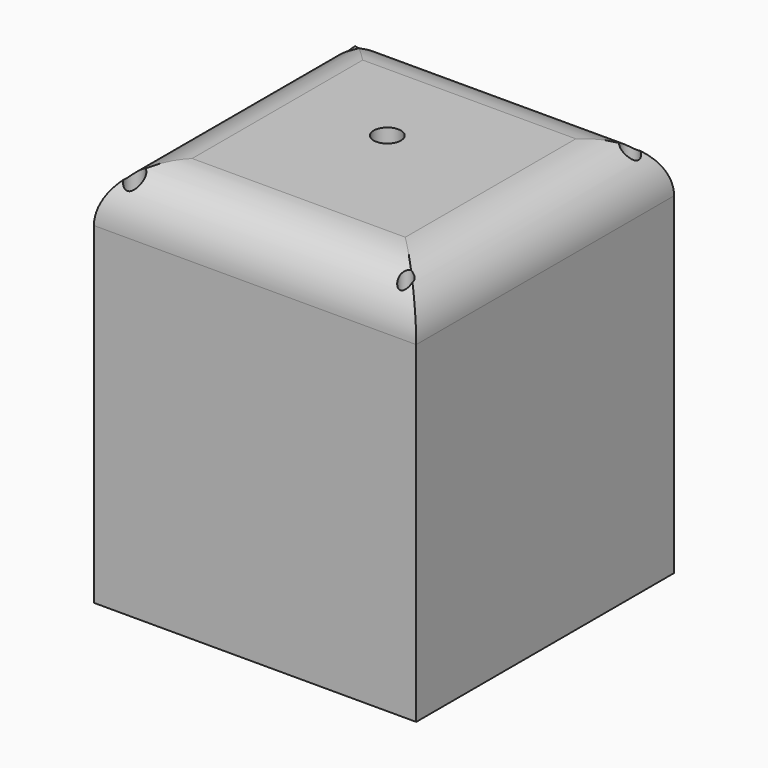
from build123d import *

# Parameters (mm, degrees)
F0_W         = 60
F0_H         = 60
F0_R         = 4
F0_R_2       = 2.5
F0_R_3       = 3.4946911037
F0_R_4       = 3.5
F1_DEPTH     = 50
F2_T1_DEPTH  = 75.4
F2_T3_DEPTH  = 25.2382554531
F2_T5_DEPTH  = 27.4689431906
F2_T7_DEPTH  = 23.1458252341
F2_T9_DEPTH  = 24.307484892
F3_W         = 60
F3_H         = 60
F3_W_2       = 50.3480000794
F3_H_2       = 50.3480000794
F4_DEPTH     = 20
F5_W         = 60
F5_H         = 60
F6_DEPTH     = 2
F7_R         = 5.1102202796
F8_DEPTH     = 70
F9_T1_DEPTH  = 50.3480000794
F9_T3_DEPTH  = 50.3480000794
F9_T7_DEPTH  = 110.8
F9_T9_DEPTH  = 110.8
F10_T1_DEPTH = 69.9999999998
F10_T4_ANGLE = 90
F11_T1_DEPTH = 69.9999999998
F11_T4_ANGLE = 90
F12_T1_DEPTH = 69.9999999998
F12_T4_ANGLE = 90
F13_T1_DEPTH = 24.2745776091
F13_T3_DEPTH = 45.7254223907
F13_T6_ANGLE = 90
F14_R        = 1.700912826
F14_R_2      = 1.2677188497
F14_R_3      = 1.5887309538
F14_R_4      = 2.5350136115
F15_DEPTH    = 72.001
F16_R        = 2.5348197432
F17_DEPTH    = 72.0010001


# Not quite as in the source:
# - a fillet or chamfer that OpenCascade refuses, or shapes differently, is made with other operations: its cross-section is extruded or revolved along the edge and cut away or added


with BuildPart() as f1:
    # F0 (on Top) → F1 (new body)
    with BuildSketch(Plane.XY):
        with Locations((-30, 30)):
            Rectangle(F0_W, F0_H)
        with Locations((-31.7886509001, 10.1095326245)):
            Circle(F0_R, mode=Mode.SUBTRACT)
        with Locations((-48.9362515509, 26.676196605)):
            Circle(F0_R_2, mode=Mode.SUBTRACT)
        Polygon((-4.8259999603, 24.6461443603), (-4.8259999603, 4.8259999603), (-22.2616568208, 4.8259999603), (-22.2616568208, 16.4334848523), (-39.9156734347, 16.4334848523), (-39.9156734347, 4.8259999603), (-55.1740000397, 4.8259999603), (-55.1740000397, 22.681651637), (-43.3133915067, 22.681651637), (-43.3133915067, 30), (-55.1740000397, 30), (-55.1740000397, 55.1740000397), (-42.5382554531, 55.1740000397), (-42.5382554531, 44.7281748056), (-30, 44.7281748056), (-30, 55.1740000397), (-4.8259999603, 55.1740000397), (-4.8259999603, 37.5920906663), (-19.5949431509, 37.5920906663), (-19.5949431509, 24.6461443603), align=None, mode=Mode.SUBTRACT)
        with Locations((-36.420982331, 50.7049895823)):
            Circle(F0_R_3, mode=Mode.SUBTRACT)
        with Locations((-12.2104715556, 31.8728536367)):
            Circle(F0_R_4, mode=Mode.SUBTRACT)
    extrude(amount=F1_DEPTH)

    # F2: fillet of radius 5.08 on 13 edges, made by hand

    # F2_s2 → F2_t1 (cut)
    with BuildSketch(Plane.XY.offset(-12.7)):
        with BuildLine():
            ThreePointArc((-43.3133915067, 24.92), (-44.8012890582, 28.5121024484), (-48.3933915067, 30))
            Line((-48.3933915067, 30), (-43.3133915067, 30))
            Line((-43.3133915067, 30), (-43.3133915067, 24.92))
        make_face()
        with BuildLine():
            ThreePointArc((-48.3933915067, 22.681651637), (-44.8012890582, 24.1695491885), (-43.3133915067, 27.761651637))
            Line((-43.3133915067, 27.761651637), (-43.3133915067, 22.681651637))
            Line((-43.3133915067, 22.681651637), (-48.3933915067, 22.681651637))
        make_face()
        with BuildLine():
            ThreePointArc((-19.5949431509, 29.7261443603), (-18.1070455993, 26.1340419119), (-14.5149431509, 24.6461443603))
            Line((-14.5149431509, 24.6461443603), (-19.5949431509, 24.6461443603))
            Line((-19.5949431509, 24.6461443603), (-19.5949431509, 29.7261443603))
        make_face()
        with BuildLine():
            ThreePointArc((-14.5149431509, 37.5920906663), (-18.1070455993, 36.1041931147), (-19.5949431509, 32.5120906663))
            Line((-19.5949431509, 32.5120906663), (-19.5949431509, 37.5920906663))
            Line((-19.5949431509, 37.5920906663), (-14.5149431509, 37.5920906663))
        make_face()
        with BuildLine():
            ThreePointArc((-34.8356734347, 16.4334848523), (-38.4277758832, 14.9455873007), (-39.9156734347, 11.3534848523))
            Line((-39.9156734347, 11.3534848523), (-39.9156734347, 16.4334848523))
            Line((-39.9156734347, 16.4334848523), (-34.8356734347, 16.4334848523))
        make_face()
        with BuildLine():
            ThreePointArc((-22.2616568208, 11.3534848523), (-23.7495543723, 14.9455873007), (-27.3416568208, 16.4334848523))
            Line((-27.3416568208, 16.4334848523), (-22.2616568208, 16.4334848523))
            Line((-22.2616568208, 16.4334848523), (-22.2616568208, 11.3534848523))
        make_face()
    extrude(amount=F2_T1_DEPTH, mode=Mode.SUBTRACT)

    # F2_s4 → F2_t3 (cut)
    with BuildSketch(Plane.YZ.offset(-42.5382554531)):
        with BuildLine():
            ThreePointArc((44.7281748056, 44.92), (46.2160723572, 48.5121024484), (49.8081748056, 50))
            Line((49.8081748056, 50), (44.7281748056, 50))
            Line((44.7281748056, 50), (44.7281748056, 44.92))
        make_face()
    extrude(amount=F2_T3_DEPTH, mode=Mode.SUBTRACT)

    # F2_s6 → F2_t5 (cut)
    with BuildSketch(Plane.YZ.offset(-32.2949431509)):
        with BuildLine():
            ThreePointArc((37.5920906663, 44.92), (36.1041931147, 48.5121024484), (32.5120906663, 50))
            Line((32.5120906663, 50), (37.5920906663, 50))
            Line((37.5920906663, 50), (37.5920906663, 44.92))
        make_face()
        with BuildLine():
            ThreePointArc((24.6461443603, 44.92), (26.1340419119, 48.5121024484), (29.7261443603, 50))
            Line((29.7261443603, 50), (24.6461443603, 50))
            Line((24.6461443603, 50), (24.6461443603, 44.92))
        make_face()
    extrude(amount=F2_T5_DEPTH, mode=Mode.SUBTRACT)

    # F2_s8 → F2_t7 (cut)
    with BuildSketch(Plane.XZ.offset(-55.1740000397)):
        with BuildLine():
            ThreePointArc((-42.5382554531, 44.92), (-41.0503579015, 48.5121024484), (-37.4582554531, 50))
            Line((-37.4582554531, 50), (-42.5382554531, 50))
            Line((-42.5382554531, 50), (-42.5382554531, 44.92))
        make_face()
        with BuildLine():
            ThreePointArc((-30, 44.92), (-31.4878975516, 48.5121024484), (-35.08, 50))
            Line((-35.08, 50), (-30, 50))
            Line((-30, 50), (-30, 44.92))
        make_face()
    extrude(amount=F2_T7_DEPTH, mode=Mode.SUBTRACT)

    # F2_s10 → F2_t9 (cut)
    with BuildSketch(Plane.XZ.offset(-29.1334848523)):
        with BuildLine():
            ThreePointArc((-22.2616568208, 44.92), (-23.7495543723, 48.5121024484), (-27.3416568208, 50))
            Line((-27.3416568208, 50), (-22.2616568208, 50))
            Line((-22.2616568208, 50), (-22.2616568208, 44.92))
        make_face()
        with BuildLine():
            ThreePointArc((-39.9156734347, 44.92), (-38.4277758832, 48.5121024484), (-34.8356734347, 50))
            Line((-34.8356734347, 50), (-39.9156734347, 50))
            Line((-39.9156734347, 50), (-39.9156734347, 44.92))
        make_face()
    extrude(amount=F2_T9_DEPTH, mode=Mode.SUBTRACT)

    # F3 (on face) → F4 (join)
    with BuildSketch(Plane.XY.offset(50)):
        with Locations((-30, 30)):
            Rectangle(F3_W, F3_H)
        with Locations((-30, 30)):
            Rectangle(F3_W_2, F3_H_2, mode=Mode.SUBTRACT)
    extrude(amount=F4_DEPTH)

    # F5 (on face) → F6 (join)
    with BuildSketch(Plane.XY.offset(70)):
        with Locations((-30, 30)):
            Rectangle(F5_W, F5_H)
    extrude(amount=F6_DEPTH)

    # F7 (on Top) → F8 (join)
    with BuildSketch(Plane.XY):
        with Locations((-32.2121977806, 33.5347950459)):
            Circle(F7_R)
    extrude(amount=F8_DEPTH)

    # F9: fillet of radius 10.16 on 9 edges, made by hand

    # F9_s2 → F9_t1 (join)
    with BuildSketch(Plane.XZ.offset(-55.1740000397)):
        with BuildLine():
            ThreePointArc((-4.8259999603, 59.84), (-7.8017950634, 67.0242048969), (-14.9859999603, 70))
            Line((-14.9859999603, 70), (-4.8259999603, 70))
            Line((-4.8259999603, 70), (-4.8259999603, 59.84))
        make_face()
        with BuildLine():
            ThreePointArc((-55.1740000397, 59.84), (-52.1982049366, 67.0242048969), (-45.0140000397, 70))
            Line((-45.0140000397, 70), (-55.1740000397, 70))
            Line((-55.1740000397, 70), (-55.1740000397, 59.84))
        make_face()
    extrude(amount=F9_T1_DEPTH)

    # F9_s4 → F9_t3 (join)
    with BuildSketch(Plane.YZ.offset(-55.1740000397)):
        with BuildLine():
            ThreePointArc((4.8259999603, 59.84), (7.8017950634, 67.0242048969), (14.9859999603, 70))
            Line((14.9859999603, 70), (4.8259999603, 70))
            Line((4.8259999603, 70), (4.8259999603, 59.84))
        make_face()
        with BuildLine():
            ThreePointArc((55.1740000397, 59.84), (52.1982049366, 67.0242048969), (45.0140000397, 70))
            Line((45.0140000397, 70), (55.1740000397, 70))
            Line((55.1740000397, 70), (55.1740000397, 59.84))
        make_face()
    extrude(amount=F9_T3_DEPTH)

    # F9_s5 → F9_t6 (revolve)
    with BuildSketch(Plane.XZ.offset(-33.5347950459)):
        with BuildLine():
            ThreePointArc((-16.941977501, 70), (-24.1261823978, 67.0242048969), (-27.101977501, 59.84))
            Line((-27.101977501, 59.84), (-27.101977501, 70))
            Line((-27.101977501, 70), (-16.941977501, 70))
        make_face()
    revolve(axis=Axis((-32.2121977806, 33.5347950459, 70), (0, 0, 1)))

    # F9_s8 → F9_t7 (cut)
    with BuildSketch(Plane.XZ.offset(-85.4)):
        with BuildLine():
            ThreePointArc((-10.16, 72), (-2.9757951031, 69.0242048969), (0, 61.84))
            Line((0, 61.84), (0, 72))
            Line((0, 72), (-10.16, 72))
        make_face()
        with BuildLine():
            ThreePointArc((-60, 61.84), (-57.0242048969, 69.0242048969), (-49.84, 72))
            Line((-49.84, 72), (-60, 72))
            Line((-60, 72), (-60, 61.84))
        make_face()
    extrude(amount=F9_T7_DEPTH, mode=Mode.SUBTRACT)

    # F9_s10 → F9_t9 (cut)
    with BuildSketch(Plane.YZ.offset(-85.4)):
        with BuildLine():
            ThreePointArc((49.84, 72), (57.0242048969, 69.0242048969), (60, 61.84))
            Line((60, 61.84), (60, 72))
            Line((60, 72), (49.84, 72))
        make_face()
        with BuildLine():
            ThreePointArc((0, 61.84), (2.9757951031, 69.0242048969), (10.16, 72))
            Line((10.16, 72), (0, 72))
            Line((0, 72), (0, 61.84))
        make_face()
    extrude(amount=F9_T9_DEPTH, mode=Mode.SUBTRACT)

    # F10: fillet of radius 12.7 on 1 edges, made by hand

    # F10_s2 → F10_t1 (join)
    with BuildSketch(Plane.XY):
        with BuildLine():
            ThreePointArc((-55.1740000397, 17.5259999603), (-51.4542561608, 8.5457438392), (-42.4740000397, 4.8259999603))
            Line((-42.4740000397, 4.8259999603), (-55.1740000397, 4.8259999603))
            Line((-55.1740000397, 4.8259999603), (-55.1740000397, 17.5259999603))
        make_face()
    extrude(amount=F10_T1_DEPTH)

    # F10_s3 → F10_t4 (revolve)
    with BuildSketch(Plane.XZ.offset(-17.5259999603)):
        with BuildLine():
            ThreePointArc((-45.0140000398, 70), (-52.1982049366, 67.0242048969), (-55.1740000397, 59.8400000002))
            Line((-55.1740000397, 59.8400000002), (-55.1740000397, 70))
            Line((-55.1740000397, 70), (-45.0140000398, 70))
        make_face()
    revolve(axis=Axis((-42.4740000397, 17.5259999603, 70), (0, 0, 1)), revolution_arc=F10_T4_ANGLE)

    # F11: fillet of radius 12.7 on 1 edges, made by hand

    # F11_s2 → F11_t1 (join)
    with BuildSketch(Plane.XY):
        with BuildLine():
            ThreePointArc((-4.8259999603, 17.5259999603), (-8.5457438392, 8.5457438392), (-17.5259999603, 4.8259999603))
            Line((-17.5259999603, 4.8259999603), (-4.8259999603, 4.8259999603))
            Line((-4.8259999603, 4.8259999603), (-4.8259999603, 17.5259999603))
        make_face()
    extrude(amount=F11_T1_DEPTH)

    # F11_s3 → F11_t4 (revolve)
    with BuildSketch(Plane.YZ.offset(-17.5259999603)):
        with BuildLine():
            ThreePointArc((14.9859999602, 70), (7.8017950634, 67.0242048969), (4.8259999603, 59.8400000002))
            Line((4.8259999603, 59.8400000002), (4.8259999603, 70))
            Line((4.8259999603, 70), (14.9859999602, 70))
        make_face()
    revolve(axis=Axis((-17.5259999603, 17.5259999603, 70), (0, 0, 1)), revolution_arc=F11_T4_ANGLE)

    # F12: fillet of radius 12.7 on 1 edges, made by hand

    # F12_s2 → F12_t1 (join)
    with BuildSketch(Plane.XY):
        with BuildLine():
            ThreePointArc((-4.8259999603, 42.4740000397), (-8.5457438392, 51.4542561608), (-17.5259999603, 55.1740000397))
            Line((-17.5259999603, 55.1740000397), (-4.8259999603, 55.1740000397))
            Line((-4.8259999603, 55.1740000397), (-4.8259999603, 42.4740000397))
        make_face()
    extrude(amount=F12_T1_DEPTH)

    # F12_s3 → F12_t4 (revolve)
    with BuildSketch(Plane.XZ.offset(-42.4740000397)):
        with BuildLine():
            ThreePointArc((-14.9859999602, 70), (-7.8017950634, 67.0242048969), (-4.8259999603, 59.8400000002))
            Line((-4.8259999603, 59.8400000002), (-4.8259999603, 70))
            Line((-4.8259999603, 70), (-14.9859999602, 70))
        make_face()
    revolve(axis=Axis((-17.5259999603, 42.4740000397, 70), (0, 0, 1)), revolution_arc=F12_T4_ANGLE)

    # F13: fillet of radius 12.7 on 1 edges, made by hand

    # F13_s2 → F13_t1 (join)
    with BuildSketch(Plane.XY.offset(45.7254223907)):
        with BuildLine():
            ThreePointArc((-55.1740000397, 42.4740000397), (-51.4542561608, 51.4542561608), (-42.4740000397, 55.1740000397))
            Line((-42.4740000397, 55.1740000397), (-55.1740000397, 55.1740000397))
            Line((-55.1740000397, 55.1740000397), (-55.1740000397, 42.4740000397))
        make_face()
    extrude(amount=F13_T1_DEPTH)

    # F13_s4 → F13_t3 (join)
    with BuildSketch(Plane.XY):
        with BuildLine():
            ThreePointArc((-55.1740000397, 42.4741625903), (-51.4769452175, 51.4316721842), (-42.5382554531, 55.1740000397))
            Line((-42.5382554531, 55.1740000397), (-55.1740000397, 55.1740000397))
            Line((-55.1740000397, 55.1740000397), (-55.1740000397, 42.4741625903))
        make_face()
    extrude(amount=F13_T3_DEPTH)

    # F13_s5 → F13_t6 (revolve)
    with BuildSketch(Plane.YZ.offset(-42.4740000397)):
        with BuildLine():
            ThreePointArc((45.0140000398, 70), (52.1982049366, 67.0242048969), (55.1740000397, 59.8400000002))
            Line((55.1740000397, 59.8400000002), (55.1740000397, 70))
            Line((55.1740000397, 70), (45.0140000398, 70))
        make_face()
    revolve(axis=Axis((-42.4740000397, 42.4740000397, 70), (0, 0, 1)), revolution_arc=F13_T6_ANGLE)

    # F14 (on face) → F15 (cut, through all)
    with BuildSketch(Plane(origin=(0, 0, 0), x_dir=(1, 0, 0), z_dir=(0, 0, -1))):
        with Locations((-55.4954074323, -3.8566410076)):
            Circle(F14_R)
        with Locations((-4.7742491588, -3.5582811106)):
            Circle(F14_R_2)
        with Locations((-4.3229921721, -55.1740000397)):
            Circle(F14_R_3)
        with Locations((-55.1740000397, -55.1740000397)):
            Circle(F14_R_4)
    extrude(amount=-F15_DEPTH, mode=Mode.SUBTRACT)

    # F16 (on face) → F17 (cut, through all)
    with BuildSketch(Plane(origin=(0, 0, 0), x_dir=(1, 0, 0), z_dir=(0, 0, -1))):
        with Locations((-32.2121977806, -33.5347950459)):
            Circle(F16_R)
    extrude(amount=-F17_DEPTH, mode=Mode.SUBTRACT)


solid = f1.part
